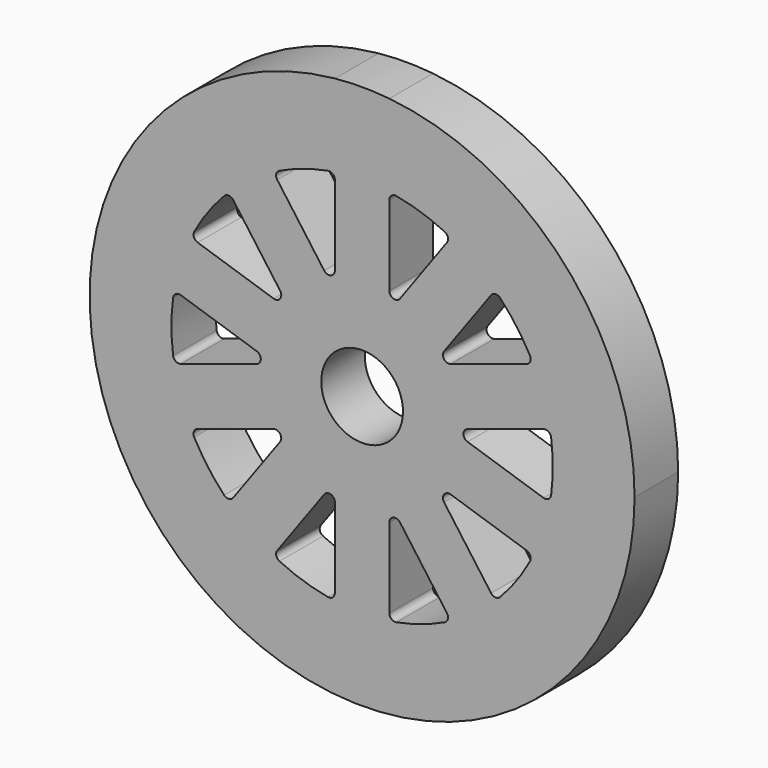
from build123d import *

# Parameters (mm, degrees)
F1_DEPTH = 1


with BuildPart() as f1:
    # F0 (on Front) → F1 (new body, symmetric)
    with BuildSketch(Plane.XZ):
        with BuildLine():
            ThreePointArc((-1, 9.949874), (-6.708204, -7.416198), (10, 0))
            ThreePointArc((10, 0), (7.416198, 6.708204), (1, 9.949874))
            ThreePointArc((1, 9.949874), (0, 10), (-1, 9.949874))
        make_face()
        with BuildLine():
            ThreePointArc((-3.033244, -6.308679), (-3.148856, -6.167132), (-3.114236, -5.987679))
            Line((-3.114236, -5.987679), (-1.389983, -3.614449))
            ThreePointArc((-1.389983, -3.614449), (-1.14896, -3.536136), (-1, -3.741162))
            Line((-1, -3.741162), (-1, -6.674636))
            ThreePointArc((-1, -6.674636), (-1.077471, -6.840166), (-1.254203, -6.886725))
            ThreePointArc((-1.254203, -6.886725), (-2.163119, -6.657396), (-3.033244, -6.308679))
        make_face(mode=Mode.SUBTRACT)
        with BuildLine():
            ThreePointArc((-6.162094, -3.320932), (-6.172427, -3.138463), (-6.038939, -3.013632))
            Line((-6.038939, -3.013632), (-3.24904, -2.107139))
            ThreePointArc((-3.24904, -2.107139), (-3.008017, -2.185452), (-3.008017, -2.438878))
            Line((-3.008017, -2.438878), (-4.73227, -4.812109))
            ThreePointArc((-4.73227, -4.812109), (-4.892241, -4.900489), (-5.062586, -4.834275))
            ThreePointArc((-5.062586, -4.834275), (-5.663119, -4.114497), (-6.162094, -3.320932))
        make_face(mode=Mode.SUBTRACT)
        with BuildLine():
            ThreePointArc((1.254203, -6.886725), (1.077471, -6.840166), (1, -6.674636))
            Line((1, -6.674636), (1, -3.741162))
            ThreePointArc((1, -3.741162), (1.14896, -3.536136), (1.389983, -3.614449))
            Line((1.389983, -3.614449), (3.114236, -5.987679))
            ThreePointArc((3.114236, -5.987679), (3.148856, -6.167132), (3.033244, -6.308679))
            ThreePointArc((3.033244, -6.308679), (2.163119, -6.657396), (1.254203, -6.886725))
        make_face(mode=Mode.SUBTRACT)
        with BuildLine():
            ThreePointArc((5.062586, -4.834275), (4.892241, -4.900489), (4.73227, -4.812109))
            Line((4.73227, -4.812109), (3.008017, -2.438878))
            ThreePointArc((3.008017, -2.438878), (3.008017, -2.185452), (3.24904, -2.107139))
            Line((3.24904, -2.107139), (6.038939, -3.013632))
            ThreePointArc((6.038939, -3.013632), (6.172427, -3.138463), (6.162094, -3.320932))
            ThreePointArc((6.162094, -3.320932), (5.663119, -4.114497), (5.062586, -4.834275))
        make_face(mode=Mode.SUBTRACT)
        with BuildLine():
            ThreePointArc((6.937234, -0.935297), (6.838341, -1.088992), (6.656973, -1.111519))
            Line((6.656973, -1.111519), (3.867074, -0.205026))
            ThreePointArc((3.867074, -0.205026), (3.718113, 0), (3.867074, 0.205026))
            Line((3.867074, 0.205026), (6.656973, 1.111519))
            ThreePointArc((6.656973, 1.111519), (6.838341, 1.088992), (6.937234, 0.935297))
            ThreePointArc((6.937234, 0.935297), (7, 0), (6.937234, -0.935297))
        make_face(mode=Mode.SUBTRACT)
        with BuildLine():
            ThreePointArc((-6.937234, -0.935297), (-7, 0), (-6.937234, 0.935297))
            ThreePointArc((-6.937234, 0.935297), (-6.838341, 1.088992), (-6.656973, 1.111519))
            Line((-6.656973, 1.111519), (-3.867074, 0.205026))
            ThreePointArc((-3.867074, 0.205026), (-3.718113, 0), (-3.867074, -0.205026))
            Line((-3.867074, -0.205026), (-6.656973, -1.111519))
            ThreePointArc((-6.656973, -1.111519), (-6.838341, -1.088992), (-6.937234, -0.935297))
        make_face(mode=Mode.SUBTRACT)
        with BuildLine():
            ThreePointArc((-5.062586, 4.834275), (-4.892241, 4.900489), (-4.73227, 4.812109))
            Line((-4.73227, 4.812109), (-3.008017, 2.438878))
            ThreePointArc((-3.008017, 2.438878), (-3.008017, 2.185452), (-3.24904, 2.107139))
            Line((-3.24904, 2.107139), (-6.038939, 3.013632))
            ThreePointArc((-6.038939, 3.013632), (-6.172427, 3.138463), (-6.162094, 3.320932))
            ThreePointArc((-6.162094, 3.320932), (-5.663119, 4.114497), (-5.062586, 4.834275))
        make_face(mode=Mode.SUBTRACT)
        with BuildLine():
            ThreePointArc((-1.254203, 6.886725), (-1.077471, 6.840166), (-1, 6.674636))
            Line((-1, 6.674636), (-1, 3.741162))
            ThreePointArc((-1, 3.741162), (-1.14896, 3.536136), (-1.389983, 3.614449))
            Line((-1.389983, 3.614449), (-3.114236, 5.987679))
            ThreePointArc((-3.114236, 5.987679), (-3.148856, 6.167132), (-3.033244, 6.308679))
            ThreePointArc((-3.033244, 6.308679), (-2.163119, 6.657396), (-1.254203, 6.886725))
        make_face(mode=Mode.SUBTRACT)
        with BuildLine():
            ThreePointArc((0, 1.5), (1.06066, 1.06066), (1.5, 0))
            ThreePointArc((1.5, 0), (-1.06066, -1.06066), (0, 1.5))
        make_face(mode=Mode.SUBTRACT)
        with BuildLine():
            ThreePointArc((6.162094, 3.320932), (6.172427, 3.138463), (6.038939, 3.013632))
            Line((6.038939, 3.013632), (3.24904, 2.107139))
            ThreePointArc((3.24904, 2.107139), (3.008017, 2.185452), (3.008017, 2.438878))
            Line((3.008017, 2.438878), (4.73227, 4.812109))
            ThreePointArc((4.73227, 4.812109), (4.892241, 4.900489), (5.062586, 4.834275))
            ThreePointArc((5.062586, 4.834275), (5.663119, 4.114497), (6.162094, 3.320932))
        make_face(mode=Mode.SUBTRACT)
        with BuildLine():
            Line((1, 3.741162), (1, 6.674636))
            ThreePointArc((1, 6.674636), (1.077471, 6.840166), (1.254203, 6.886725))
            ThreePointArc((1.254203, 6.886725), (2.163119, 6.657396), (3.033244, 6.308679))
            ThreePointArc((3.033244, 6.308679), (3.148856, 6.167132), (3.114236, 5.987679))
            Line((3.114236, 5.987679), (1.389983, 3.614449))
            ThreePointArc((1.389983, 3.614449), (1.14896, 3.536136), (1, 3.741162))
        make_face(mode=Mode.SUBTRACT)
    extrude(amount=F1_DEPTH, both=True)


solid = f1.part
